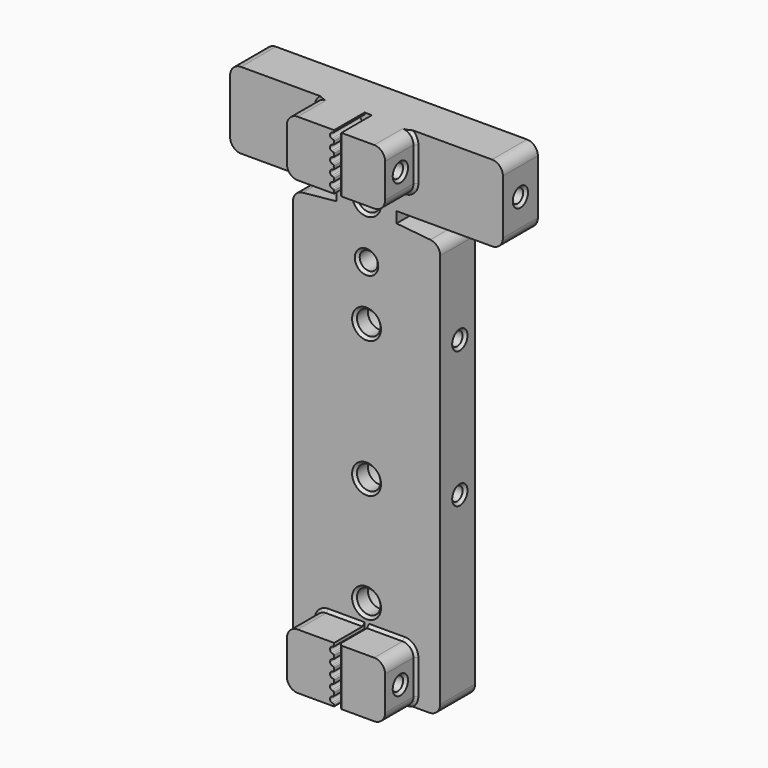
from build123d import *

# Parameters (mm, degrees)
F0_R      = 2.15
F0_R_2    = 1.65
F1_DEPTH  = 4
F3_DEPTH  = 7
F4_R      = 1.25
F5_DEPTH  = 50.001
F6_R      = 1.25
F7_DEPTH  = 13.5
F8_R      = 3.25
F9_DEPTH  = 5
F10_R     = 1.65
F11_DEPTH = 2.4
F12_R     = 2
F13_R     = 1.25
F14_DEPTH = 8.524
F15_SIZE  = 0.5


with BuildPart() as f1:
    # F0 (on Front) → F1 (new body, symmetric)
    with BuildSketch(Plane.XZ):
        Polygon((-13.5, -86), (13.5, -86), (13.5, -9.8), (5.5, -9), (5.5, -7), (13.5, -7), (25, -7), (25, 7), (-25, 7), (-25, -7), (-13.5, -7), (-5.5, -7), (-5.5, -9), (-13.5, -9.8), align=None)
        with Locations((0, -72)):
            Circle(F0_R, mode=Mode.SUBTRACT)
        with Locations((0, -52)):
            Circle(F0_R, mode=Mode.SUBTRACT)
        with Locations((0, -27)):
            Circle(F0_R, mode=Mode.SUBTRACT)
        with Locations((0, -17)):
            Circle(F0_R_2, mode=Mode.SUBTRACT)
        with Locations((0, -7)):
            Circle(F0_R, mode=Mode.SUBTRACT)
    extrude(amount=F1_DEPTH, both=True)

    # F2 (on face) → F3 (join)
    with BuildSketch(Plane.XZ.offset(4)):
        Polygon((9, 7), (0.476, 7), (0.476, 6), (0.476, 5), (0.476, 4), (0.476, 3), (0.476, 2), (0.476, 1), (0.476, 0), (0.476, -1), (0.476, -2), (0.476, -3), (0.476, -3.2598245749), (9, -3.2598245749), align=None)
        with BuildLine():
            Line((-0.354, 6.7401754251), (-0.354, 7))
            Line((-0.354, 7), (-9, 7))
            Line((-9, 7), (-9, -3.2598245749))
            Line((-9, -3.2598245749), (-0.354, -3.2598245749))
            Line((-0.354, -3.2598245749), (-0.354, -3))
            Line((-0.354, -3), (-0.354, -2.7401754251))
            ThreePointArc((-0.354, -2.7401754251), (-0.3912285883, -2.6412683541), (-0.4844347826, -2.5914568914))
            ThreePointArc((-0.4844347826, -2.5914568914), (-0.642062154, -2.5576117143), (-0.7922022472, -2.4988764045))
            ThreePointArc((-0.7922022472, -2.4988764045), (-1.0196390587, -2.2941494117), (-1.104, -2))
            ThreePointArc((-1.104, -2), (-1.0196390587, -1.7058505883), (-0.7922022472, -1.5011235955))
            ThreePointArc((-0.7922022472, -1.5011235955), (-0.642062154, -1.4423882857), (-0.4844347826, -1.4085431086))
            ThreePointArc((-0.4844347826, -1.4085431086), (-0.3912285883, -1.3587316459), (-0.354, -1.2598245749))
            Line((-0.354, -1.2598245749), (-0.354, -1))
            Line((-0.354, -1), (-0.354, -0.7401754251))
            ThreePointArc((-0.354, -0.7401754251), (-0.3912285883, -0.6412683541), (-0.4844347826, -0.5914568914))
            ThreePointArc((-0.4844347826, -0.5914568914), (-0.642062154, -0.5576117143), (-0.7922022472, -0.4988764045))
            ThreePointArc((-0.7922022472, -0.4988764045), (-1.0196390587, -0.2941494117), (-1.104, 0))
            ThreePointArc((-1.104, 0), (-1.0196390587, 0.2941494117), (-0.7922022472, 0.4988764045))
            ThreePointArc((-0.7922022472, 0.4988764045), (-0.642062154, 0.5576117143), (-0.4844347826, 0.5914568914))
            ThreePointArc((-0.4844347826, 0.5914568914), (-0.3912285883, 0.6412683541), (-0.354, 0.7401754251))
            Line((-0.354, 0.7401754251), (-0.354, 1))
            Line((-0.354, 1), (-0.354, 1.2598245749))
            ThreePointArc((-0.354, 1.2598245749), (-0.3912285883, 1.3587316459), (-0.4844347826, 1.4085431086))
            ThreePointArc((-0.4844347826, 1.4085431086), (-0.642062154, 1.4423882857), (-0.7922022472, 1.5011235955))
            ThreePointArc((-0.7922022472, 1.5011235955), (-1.0196390587, 1.7058505883), (-1.104, 2))
            ThreePointArc((-1.104, 2), (-1.0196390587, 2.2941494117), (-0.7922022472, 2.4988764045))
            ThreePointArc((-0.7922022472, 2.4988764045), (-0.642062154, 2.5576117143), (-0.4844347826, 2.5914568914))
            ThreePointArc((-0.4844347826, 2.5914568914), (-0.3912285883, 2.6412683541), (-0.354, 2.7401754251))
            Line((-0.354, 2.7401754251), (-0.354, 3))
            Line((-0.354, 3), (-0.354, 3.2598245749))
            ThreePointArc((-0.354, 3.2598245749), (-0.3912285883, 3.3587316459), (-0.4844347826, 3.4085431086))
            ThreePointArc((-0.4844347826, 3.4085431086), (-0.642062154, 3.4423882857), (-0.7922022472, 3.5011235955))
            ThreePointArc((-0.7922022472, 3.5011235955), (-1.0196390587, 3.7058505883), (-1.104, 4))
            ThreePointArc((-1.104, 4), (-1.0196390587, 4.2941494117), (-0.7922022472, 4.4988764045))
            ThreePointArc((-0.7922022472, 4.4988764045), (-0.642062154, 4.5576117143), (-0.4844347826, 4.5914568914))
            ThreePointArc((-0.4844347826, 4.5914568914), (-0.3912285883, 4.6412683541), (-0.354, 4.7401754251))
            Line((-0.354, 4.7401754251), (-0.354, 5))
            Line((-0.354, 5), (-0.354, 5.2598245749))
            ThreePointArc((-0.354, 5.2598245749), (-0.3912285883, 5.3587316459), (-0.4844347826, 5.4085431086))
            ThreePointArc((-0.4844347826, 5.4085431086), (-0.642062154, 5.4423882857), (-0.7922022472, 5.5011235955))
            ThreePointArc((-0.7922022472, 5.5011235955), (-1.0196390587, 5.7058505883), (-1.104, 6))
            ThreePointArc((-1.104, 6), (-1.0196390587, 6.2941494117), (-0.7922022472, 6.4988764045))
            ThreePointArc((-0.7922022472, 6.4988764045), (-0.642062154, 6.5576117143), (-0.4844347826, 6.5914568914))
            ThreePointArc((-0.4844347826, 6.5914568914), (-0.3912285883, 6.6412683541), (-0.354, 6.7401754251))
        make_face()
        with BuildLine():
            Line((-0.354, -84), (-0.354, -83.7401754251))
            ThreePointArc((-0.354, -83.7401754251), (-0.3912285883, -83.6412683541), (-0.4844347826, -83.5914568914))
            ThreePointArc((-0.4844347826, -83.5914568914), (-0.642062154, -83.5576117143), (-0.7922022472, -83.4988764045))
            ThreePointArc((-0.7922022472, -83.4988764045), (-1.0196390587, -83.2941494117), (-1.104, -83))
            ThreePointArc((-1.104, -83), (-1.0196390587, -82.7058505883), (-0.7922022472, -82.5011235955))
            ThreePointArc((-0.7922022472, -82.5011235955), (-0.642062154, -82.4423882857), (-0.4844347826, -82.4085431086))
            ThreePointArc((-0.4844347826, -82.4085431086), (-0.3912285883, -82.3587316459), (-0.354, -82.2598245749))
            Line((-0.354, -82.2598245749), (-0.354, -82))
            Line((-0.354, -82), (-0.354, -81.7401754251))
            ThreePointArc((-0.354, -81.7401754251), (-0.3912285883, -81.6412683541), (-0.4844347826, -81.5914568914))
            ThreePointArc((-0.4844347826, -81.5914568914), (-0.642062154, -81.5576117143), (-0.7922022472, -81.4988764045))
            ThreePointArc((-0.7922022472, -81.4988764045), (-1.0196390587, -81.2941494117), (-1.104, -81))
            ThreePointArc((-1.104, -81), (-1.0196390587, -80.7058505883), (-0.7922022472, -80.5011235955))
            ThreePointArc((-0.7922022472, -80.5011235955), (-0.642062154, -80.4423882857), (-0.4844347826, -80.4085431086))
            ThreePointArc((-0.4844347826, -80.4085431086), (-0.3912285883, -80.3587316459), (-0.354, -80.2598245749))
            Line((-0.354, -80.2598245749), (-0.354, -80))
            Line((-0.354, -80), (-0.354, -79.7401754251))
            ThreePointArc((-0.354, -79.7401754251), (-0.3912285883, -79.6412683541), (-0.4844347826, -79.5914568914))
            ThreePointArc((-0.4844347826, -79.5914568914), (-0.642062154, -79.5576117143), (-0.7922022472, -79.4988764045))
            ThreePointArc((-0.7922022472, -79.4988764045), (-1.0196390587, -79.2941494117), (-1.104, -79))
            ThreePointArc((-1.104, -79), (-1.0196390587, -78.7058505883), (-0.7922022472, -78.5011235955))
            ThreePointArc((-0.7922022472, -78.5011235955), (-0.642062154, -78.4423882857), (-0.4844347826, -78.4085431086))
            ThreePointArc((-0.4844347826, -78.4085431086), (-0.3912285883, -78.3587316459), (-0.354, -78.2598245749))
            Line((-0.354, -78.2598245749), (-0.354, -78))
            Line((-0.354, -78), (-0.354, -77.7401754251))
            ThreePointArc((-0.354, -77.7401754251), (-0.3912285883, -77.6412683541), (-0.4844347826, -77.5914568914))
            ThreePointArc((-0.4844347826, -77.5914568914), (-0.642062154, -77.5576117143), (-0.7922022472, -77.4988764045))
            ThreePointArc((-0.7922022472, -77.4988764045), (-1.0196390587, -77.2941494117), (-1.104, -77))
            ThreePointArc((-1.104, -77), (-1.0196390587, -76.7058505883), (-0.7922022472, -76.5011235955))
            ThreePointArc((-0.7922022472, -76.5011235955), (-0.642062154, -76.4423882857), (-0.4844347826, -76.4085431086))
            ThreePointArc((-0.4844347826, -76.4085431086), (-0.3912285883, -76.3587316459), (-0.354, -76.2598245749))
            Line((-0.354, -76.2598245749), (-0.354, -76))
            Line((-0.354, -76), (-0.354, -75.7401754251))
            Line((-0.354, -75.7401754251), (-9, -75.7401754251))
            Line((-9, -75.7401754251), (-9, -86))
            Line((-9, -86), (-0.354, -86))
            Line((-0.354, -86), (-0.354, -85.7401754251))
            ThreePointArc((-0.354, -85.7401754251), (-0.3912285883, -85.6412683541), (-0.4844347826, -85.5914568914))
            ThreePointArc((-0.4844347826, -85.5914568914), (-0.642062154, -85.5576117143), (-0.7922022472, -85.4988764045))
            ThreePointArc((-0.7922022472, -85.4988764045), (-1.0196390587, -85.2941494117), (-1.104, -85))
            ThreePointArc((-1.104, -85), (-1.0196390587, -84.7058505883), (-0.7922022472, -84.5011235955))
            ThreePointArc((-0.7922022472, -84.5011235955), (-0.642062154, -84.4423882857), (-0.4844347826, -84.4085431086))
            ThreePointArc((-0.4844347826, -84.4085431086), (-0.3912285883, -84.3587316459), (-0.354, -84.2598245749))
            Line((-0.354, -84.2598245749), (-0.354, -84))
        make_face()
        Polygon((0.476, -75.7401754251), (0.476, -76), (0.476, -77), (0.476, -78), (0.476, -79), (0.476, -80), (0.476, -81), (0.476, -82), (0.476, -83), (0.476, -84), (0.476, -85), (0.476, -86), (9, -86), (9, -75.7401754251), align=None)
    extrude(amount=F3_DEPTH)

    # F4 (on face) → F5 (cut, through all)
    with BuildSketch(Plane.YZ.offset(25)):
        Circle(F4_R)
    extrude(amount=-F5_DEPTH, mode=Mode.SUBTRACT)

    # F6 (on face) → F7 (cut)
    with BuildSketch(Plane.YZ.offset(13.5)):
        with Locations((0.5, -27)):
            Circle(F6_R)
        with Locations((0.5, -52)):
            Circle(F6_R)
    extrude(amount=-F7_DEPTH, mode=Mode.SUBTRACT)

    # F8 (on face) → F9 (cut)
    with BuildSketch(Plane(origin=(0, 4, 0), x_dir=(-1, 0, 0), z_dir=(0, 1, 0))):
        with Locations((0, -7)):
            Circle(F8_R)
        with Locations((0, -27)):
            Circle(F8_R)
        with Locations((0, -52)):
            Circle(F8_R)
        with Locations((0, -72)):
            Circle(F8_R)
    extrude(amount=-F9_DEPTH, mode=Mode.SUBTRACT)

    # F10 (on face) → F11 (cut)
    with BuildSketch(Plane(origin=(0, 4, 0), x_dir=(-1, 0, 0), z_dir=(0, 1, 0))):
        Polygon((-1.6454482672, -14.15), (-3.2908965344, -17), (-1.6454482672, -19.85), (1.6454482672, -19.85), (3.2908965344, -17), (1.6454482672, -14.15), align=None)
        with Locations((0, -17)):
            Circle(F10_R, mode=Mode.SUBTRACT)
    extrude(amount=-F11_DEPTH, mode=Mode.SUBTRACT)

    # F12
    f12_edges = [f1.edges().sort_by_distance(p)[0] for p in [
        (-13.5, 0, -86),
        (13.5, 0, -86),
        (9, -7.5, -86),
        (-9, -7.5, -86),
        (9, -7.5, -3.259825),
        (-9, -7.5, -3.259825),
        (25, 0, -7),
        (9, -7.5, -75.740175),
        (-9, -7.5, -75.740175),
        (-25, 0, -7),
        (-25, 0, 7),
        (25, 0, 7),
        (9, -7.5, 7),
        (-9, -7.5, 7),
        (-13.5, 0, -9.8),
        (13.5, 0, -9.8),
    ]]
    fillet(f12_edges, radius=F12_R)

    # F13 (on face) → F14 (cut, through all)
    with BuildSketch(Plane.YZ.offset(9)):
        with Locations((-7.5, 1.8700877125)):
            Circle(F13_R)
        with Locations((-7.5, -80.8700877125)):
            Circle(F13_R)
    extrude(amount=-F14_DEPTH, mode=Mode.SUBTRACT)

    # F15 (call 1 of 19: OpenCascade refuses the feature's edges together)
    f15_edges = [f1.edges().sort_by_distance(p)[0] for p in [
        (-25, -1.25, 0),
    ]]
    chamfer(f15_edges, length=F15_SIZE)

    # F15#2 (call 2 of 19)
    f15_2_edges = [f1.edges().sort_by_distance(p)[0] for p in [
        (25, -1.25, 0),
    ]]
    chamfer(f15_2_edges, length=F15_SIZE)

    # F15#3 (call 3 of 19)
    f15_3_edges = [f1.edges().sort_by_distance(p)[0] for p in [
        (9, -8.75, 1.870088),
    ]]
    chamfer(f15_3_edges, length=F15_SIZE)

    # F15#4 (call 4 of 19)
    f15_4_edges = [f1.edges().sort_by_distance(p)[0] for p in [
        (13.5, -0.75, -27),
    ]]
    chamfer(f15_4_edges, length=F15_SIZE)

    # F15#5 (call 5 of 19)
    f15_5_edges = [f1.edges().sort_by_distance(p)[0] for p in [
        (13.5, -0.75, -52),
    ]]
    chamfer(f15_5_edges, length=F15_SIZE)

    # F15#6 (call 6 of 19)
    f15_6_edges = [f1.edges().sort_by_distance(p)[0] for p in [
        (9, -8.75, -80.870088),
    ]]
    chamfer(f15_6_edges, length=F15_SIZE)

    # F15#7 (call 7 of 19)
    f15_7_edges = [f1.edges().sort_by_distance(p)[0] for p in [
        (0.476, -11, 1.870088),
        (0.476, -7.5, 7),
    ]]
    chamfer(f15_7_edges, length=F15_SIZE)

    # F15#8 (call 8 of 19)
    f15_8_edges = [f1.edges().sort_by_distance(p)[0] for p in [
        (0.476, -8.75, 1.870088),
    ]]
    chamfer(f15_8_edges, length=F15_SIZE)

    # F15#9 (call 9 of 19)
    f15_9_edges = [f1.edges().sort_by_distance(p)[0] for p in [
        (0.476, -7.5, -86),
        (0.476, -11, -80.870088),
    ]]
    chamfer(f15_9_edges, length=F15_SIZE)

    # F15#10 (call 10 of 19)
    f15_10_edges = [f1.edges().sort_by_distance(p)[0] for p in [
        (0.476, -8.75, -80.870088),
    ]]
    chamfer(f15_10_edges, length=F15_SIZE)

    # F15#11 (call 11 of 19)
    f15_11_edges = [f1.edges().sort_by_distance(p)[0] for p in [
        (-2.15, -4, -7),
    ]]
    chamfer(f15_11_edges, length=F15_SIZE)

    # F15#12 (call 12 of 19)
    f15_12_edges = [f1.edges().sort_by_distance(p)[0] for p in [
        (-1.65, -4, -17),
    ]]
    chamfer(f15_12_edges, length=F15_SIZE)

    # F15#13 (call 13 of 19)
    f15_13_edges = [f1.edges().sort_by_distance(p)[0] for p in [
        (-2.15, -4, -27),
    ]]
    chamfer(f15_13_edges, length=F15_SIZE)

    # F15#14 (call 14 of 19)
    f15_14_edges = [f1.edges().sort_by_distance(p)[0] for p in [
        (-2.15, -4, -52),
    ]]
    chamfer(f15_14_edges, length=F15_SIZE)

    # F15#15 (call 15 of 19)
    f15_15_edges = [f1.edges().sort_by_distance(p)[0] for p in [
        (-2.15, -4, -72),
    ]]
    chamfer(f15_15_edges, length=F15_SIZE)

    # F15#16 (call 16 of 19)
    f15_16_edges = [f1.edges().sort_by_distance(p)[0] for p in [
        (8.414214, -4, 6.414214),
        (9, -4, 1.870088),
        (8.414214, -4, -2.674038),
        (3.738, -4, -3.259825),
    ]]
    chamfer(f15_16_edges, length=F15_SIZE)

    # F15#17 (call 17 of 19)
    f15_17_edges = [f1.edges().sort_by_distance(p)[0] for p in [
        (-8.414214, -4, -2.674038),
        (-3.677, -4, -3.259825),
        (-9, -4, 1.870088),
        (-8.414214, -4, 6.414214),
    ]]
    chamfer(f15_17_edges, length=F15_SIZE)

    # F15#18 (call 18 of 19)
    f15_18_edges = [f1.edges().sort_by_distance(p)[0] for p in [
        (-8.414214, -4, -76.325962),
        (-8.414214, -4, -85.414214),
        (-9, -4, -80.870088),
        (-3.677, -4, -75.740175),
    ]]
    chamfer(f15_18_edges, length=F15_SIZE)

    # F15#19 (call 19 of 19)
    f15_19_edges = [f1.edges().sort_by_distance(p)[0] for p in [
        (8.414214, -4, -76.325962),
        (3.738, -4, -75.740175),
        (9, -4, -80.870088),
        (8.414214, -4, -85.414214),
    ]]
    chamfer(f15_19_edges, length=F15_SIZE)


solid = f1.part
